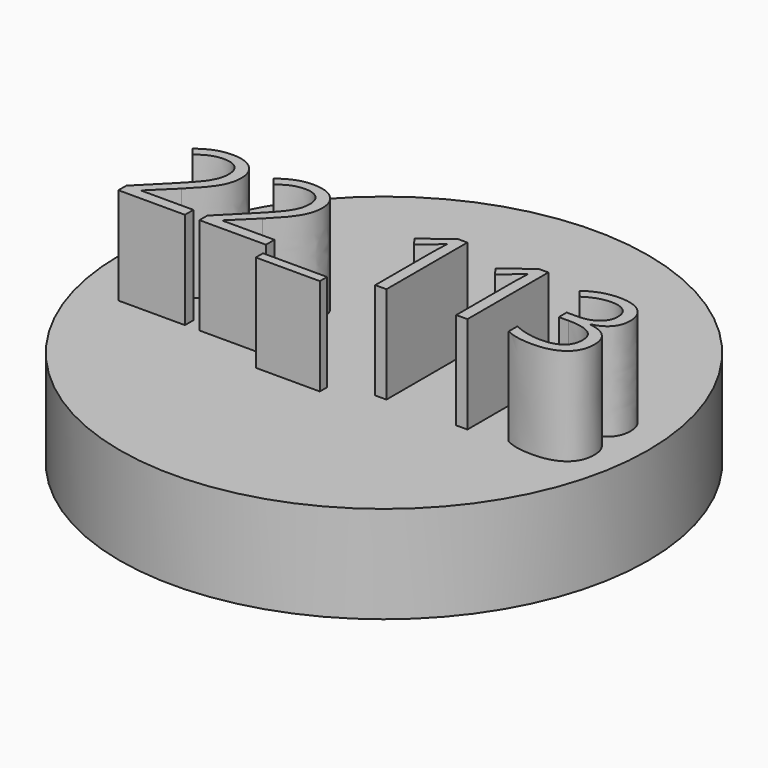
from build123d import *

# Parameters (mm, degrees)
F0_R         = 69.0483322289
F1_DEPTH     = 25.4
F2_TEXT_SIZE = 37.0363252134
F3_DEPTH     = 25.4


# Not quite as in the source:
# - Text() gives the source's letters only with a copy of the font that has no kerning and outlines rounded to 1/6400 em; it was checked with that copy


with BuildPart() as f1:
    # F0 (on Top) → F1 (new body)
    with BuildSketch(Plane.XY):
        Circle(F0_R)
    extrude(amount=F1_DEPTH)

    # F2 (on face) → F3 (join)
    with BuildSketch(Plane.XY.offset(25.4)):
        with Locations((-58.5521124303, -15.8616527915)):
            Text('22_113', F2_TEXT_SIZE, font='Open Sans', text_align=(TextAlign.LEFT, TextAlign.BOTTOM))
    extrude(amount=F3_DEPTH)


solid = f1.part
